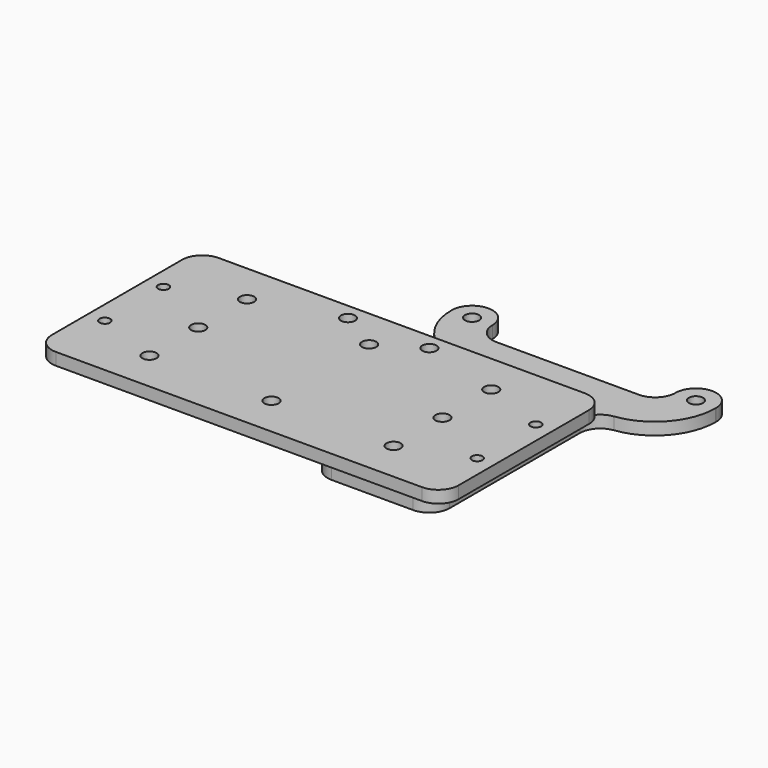
from build123d import *

# Parameters (mm, degrees)
F1_R        = 1.75
F1_R_2      = 1.3
F2_DEPTH    = 3
F3_R        = 1.75
F3_R_2      = 1.5
F4_DEPTH    = 3
F5_R        = 4.99999
F6_T1_DEPTH = 77.2156800691
F7_R        = 5
F8_R        = 2


# Not quite as in the source:
# - a fillet or chamfer that OpenCascade refuses, or shapes differently, is made with other operations: its cross-section is extruded or revolved along the edge and cut away or added
# - a fillet or chamfer is up to 0.001 mm smaller than in the source, because OpenCascade refuses the exact size
# - a feature names something its author has since deleted; it is built from what else it names


with BuildPart() as f2:
    # F1 (on offset) → F2 (new body)
    with BuildSketch(Plane.XY.offset(30)):
        Polygon((50, 25), (-50, 25), (-50, 0), (-50, -25), (50, -25), (50, 0), align=None)
        with Locations((-30, -15)):
            Circle(F1_R, mode=Mode.SUBTRACT)
        with Locations((-45.75, -9)):
            Circle(F1_R_2, mode=Mode.SUBTRACT)
        with Locations((0, -15)):
            Circle(F1_R, mode=Mode.SUBTRACT)
        with Locations((30, -15)):
            Circle(F1_R, mode=Mode.SUBTRACT)
        with Locations((45.75, -9)):
            Circle(F1_R_2, mode=Mode.SUBTRACT)
        with Locations((-30, 0)):
            Circle(F1_R, mode=Mode.SUBTRACT)
        with Locations((-45.75, 9)):
            Circle(F1_R_2, mode=Mode.SUBTRACT)
        with Locations((-30, 15)):
            Circle(F1_R, mode=Mode.SUBTRACT)
        with Locations((-10, 21)):
            Circle(F1_R, mode=Mode.SUBTRACT)
        with Locations((30, 0)):
            Circle(F1_R, mode=Mode.SUBTRACT)
        with Locations((45.75, 9)):
            Circle(F1_R_2, mode=Mode.SUBTRACT)
        with Locations((0, 15)):
            Circle(F1_R, mode=Mode.SUBTRACT)
        with Locations((10, 21)):
            Circle(F1_R, mode=Mode.SUBTRACT)
        with Locations((30, 15)):
            Circle(F1_R, mode=Mode.SUBTRACT)
    extrude(amount=F2_DEPTH)

    # F7
    f7_edges = [f2.edges().sort_by_distance(p)[0] for p in [
        (-50, 25, 31.5),
        (-50, -25, 31.5),
        (50, -25, 31.5),
        (50, 25, 31.5),
    ]]
    fillet(f7_edges, radius=F7_R)


with BuildPart() as f4:
    # F3 (on Top) → F4 (new body)
    with BuildSketch(Plane.XY):
        Polygon((-15, 66), (-15, 16), (15, 16), (15, 66), (32.5, 66), (32.5, 86), (22.5, 86), (22.5, 76), (-22.5, 76), (-22.5, 86), (-32.5, 86), (-32.5, 66), align=None)
        with Locations((-10, 21)):
            Circle(F3_R, mode=Mode.SUBTRACT)
        with Locations((10, 21)):
            Circle(F3_R, mode=Mode.SUBTRACT)
        Polygon((-10, 56.5), (-10, 66), (10, 66), (10, 56.5), (10, 50.5), (10, 26), (-10, 26), (-10, 50.5), align=None, mode=Mode.SUBTRACT)
        with Locations((-27.5, 81)):
            Circle(F3_R, mode=Mode.SUBTRACT)
        with Locations((27.5, 81)):
            Circle(F3_R, mode=Mode.SUBTRACT)
        with BuildLine():
            Line((-4.3084219849, 56.5), (-10, 56.5))
            Line((-10, 56.5), (-10, 50.5))
            Line((-10, 50.5), (-4.3084219849, 50.5))
            ThreePointArc((-4.3084219849, 50.5), (0, 48.25), (4.3084219849, 50.5))
            Line((4.3084219849, 50.5), (10, 50.5))
            Line((10, 50.5), (10, 56.5))
            Line((10, 56.5), (4.3084219849, 56.5))
            ThreePointArc((4.3084219849, 56.5), (0, 58.75), (-4.3084219849, 56.5))
        make_face()
        with Locations((-6.75, 53.5)):
            Circle(F3_R_2, mode=Mode.SUBTRACT)
        with Locations((6.75, 53.5)):
            Circle(F3_R_2, mode=Mode.SUBTRACT)
    extrude(amount=F4_DEPTH)

    # F5 (radius 5 in the source; OpenCascade refuses exactly that, so slightly less here)
    f5_edges = [f4.edges().sort_by_distance(p)[0] for p in [
        (-15, 66, 1.5),
        (-22.5, 76, 1.5),
        (-22.5, 86, 1.5),
        (-32.5, 86, 1.5),
        (22.5, 76, 1.5),
        (22.5, 86, 1.5),
        (32.5, 86, 1.5),
        (15, 66, 1.5),
        (15, 16, 1.5),
        (-15, 16, 1.5),
        (-10, 66, 1.5),
        (10, 66, 1.5),
        (10, 26, 1.5),
        (-10, 26, 1.5),
    ]]
    fillet(f5_edges, radius=F5_R)

    # F6: fillet of radius 15 on 2 edges, made by hand

    # F6_s2 → F6_t1 (cut)
    with BuildSketch(Plane.XY.offset(-37.1078400345)):
        with BuildLine():
            ThreePointArc((19.3749934375, 65.9607840623), (28.7499978125, 70.9215661169), (32.5, 80.8431360138))
            Line((32.5, 80.8431360138), (34, 80.8431360138))
            Line((34, 80.8431360138), (34, 66))
            Line((34, 66), (32.5, 64.5))
            ThreePointArc((32.5, 64.5), (19.99999, 64.5), (19.5624927812, 64.4725488671))
            Line((19.5624927812, 64.4725488671), (19.3749934375, 65.9607840623))
        make_face()
        with BuildLine():
            ThreePointArc((-19.3749934375, 65.9607840623), (-28.7499978125, 70.9215661169), (-32.5, 80.8431360138))
            Line((-32.5, 80.8431360138), (-34, 80.8431360138))
            Line((-34, 80.8431360138), (-34, 66))
            Line((-34, 66), (-32.5, 64.5))
            ThreePointArc((-32.5, 64.5), (-19.99999, 64.5), (-19.5624927812, 64.4725488671))
            Line((-19.5624927812, 64.4725488671), (-19.3749934375, 65.9607840623))
        make_face()
    extrude(amount=F6_T1_DEPTH, mode=Mode.SUBTRACT)

    # F8
    f8_edges = [f4.edges().sort_by_distance(p)[0] for p in [
        (-10, 56.5, 1.5),
        (-10, 50.5, 1.5),
        (10, 50.5, 1.5),
        (10, 56.5, 1.5),
        (4.308422, 56.5, 1.5),
        (-4.308422, 56.5, 1.5),
        (-4.308422, 50.5, 1.5),
        (4.308422, 50.5, 1.5),
    ]]
    fillet(f8_edges, radius=F8_R)


solid = Compound([f2.part, f4.part])
